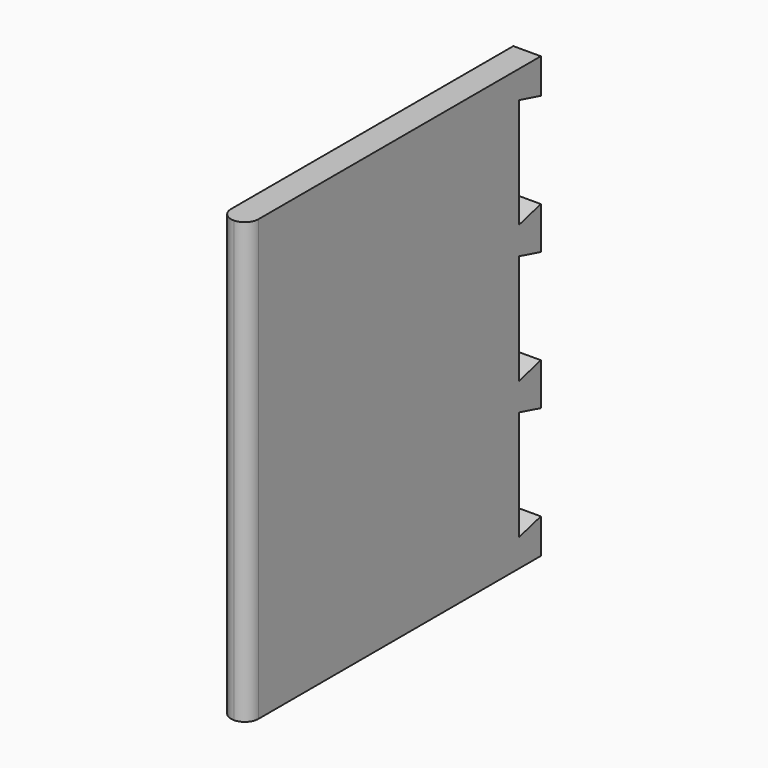
from build123d import *

# Parameters (mm, degrees)
F0_W     = 254
F0_H     = 304.8
F1_DEPTH = 9.525
F2_R     = 9.52499
F4_DEPTH = 19.051


# Not quite as in the source:
# - a fillet or chamfer is up to 0.001 mm smaller than in the source, because OpenCascade refuses the exact size
# - a feature names something its author has since deleted; it is built from what else it names


with BuildPart() as f1:
    # F0 (on Right) → F1 (new body, symmetric)
    with BuildSketch(Plane.YZ):
        Rectangle(F0_W, F0_H)
    extrude(amount=F1_DEPTH, both=True)

    # F2 (radius 9.525 in the source; OpenCascade refuses exactly that, so slightly less here)
    f2_edges = [f1.edges().sort_by_distance(p)[0] for p in [
        (9.525, -127, 0),
        (-9.525, -127, 0),
    ]]
    fillet(f2_edges, radius=F2_R)

    # F3 (on face) → F4 (cut, through all)
    with BuildSketch(Plane.YZ.offset(9.525)):
        Polygon((107.95, 57.15), (127, 62.2544321158), (127, 128.2455678842), (107.95, 133.35), align=None)
        Polygon((127, -32.9955678842), (127, 32.9955678842), (107.95, 38.1), (107.95, -38.1), align=None)
        Polygon((127, -128.2455678842), (127, -62.2544321158), (107.95, -57.15), (107.95, -133.35), align=None)
    extrude(amount=-F4_DEPTH, mode=Mode.SUBTRACT)


solid = f1.part
